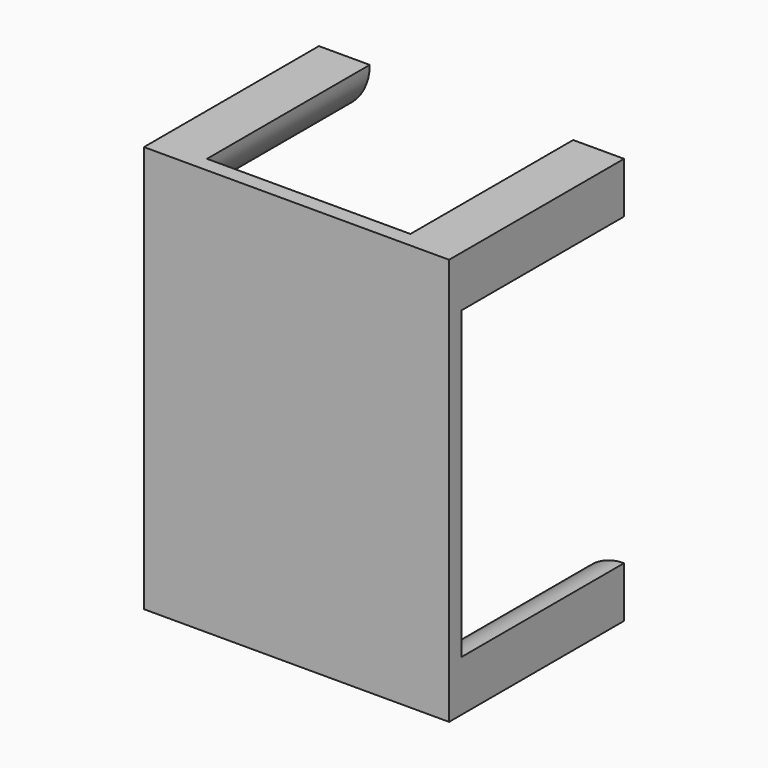
from build123d import *

# Parameters (mm, degrees)
F0_W     = 76.2
F0_H     = 101.6
F1_DEPTH = 3.81
F2_W     = 12.7
F2_H     = 12.7
F3_DEPTH = 50.8
F4_R     = 12.69999


# Not quite as in the source:
# - a fillet or chamfer is up to 0.001 mm smaller than in the source, because OpenCascade refuses the exact size


with BuildPart() as f1:
    # F0 (on Front) → F1 (new body)
    with BuildSketch(Plane.XZ):
        with Locations((4.643493332, 0.4188035619)):
            Rectangle(F0_W, F0_H)
    extrude(amount=F1_DEPTH)

    # F2 (on face) → F3 (join)
    with BuildSketch(Plane(origin=(0, 0, 0), x_dir=(-1, 0, 0), z_dir=(0, 1, 0))):
        with Locations((27.106506668, -44.0311964381)):
            Rectangle(F2_W, F2_H)
        with Locations((-36.393493332, 44.8688035619)):
            Rectangle(F2_W, F2_H)
        with Locations((27.106506668, 44.8688035619)):
            Rectangle(F2_W, F2_H)
        with Locations((-36.393493332, -44.0311964381)):
            Rectangle(F2_W, F2_H)
    extrude(amount=F3_DEPTH)

    # F4 (radius 12.7 in the source; OpenCascade refuses exactly that, so slightly less here)
    f4_edges = [f1.edges().sort_by_distance(p)[0] for p in [
        (-20.756507, 25.4, 38.518804),
        (-20.756507, 25.4, -37.681196),
        (30.043493, 25.4, -37.681196),
        (30.043493, 25.4, 38.518804),
    ]]
    fillet(f4_edges, radius=F4_R)


solid = f1.part
